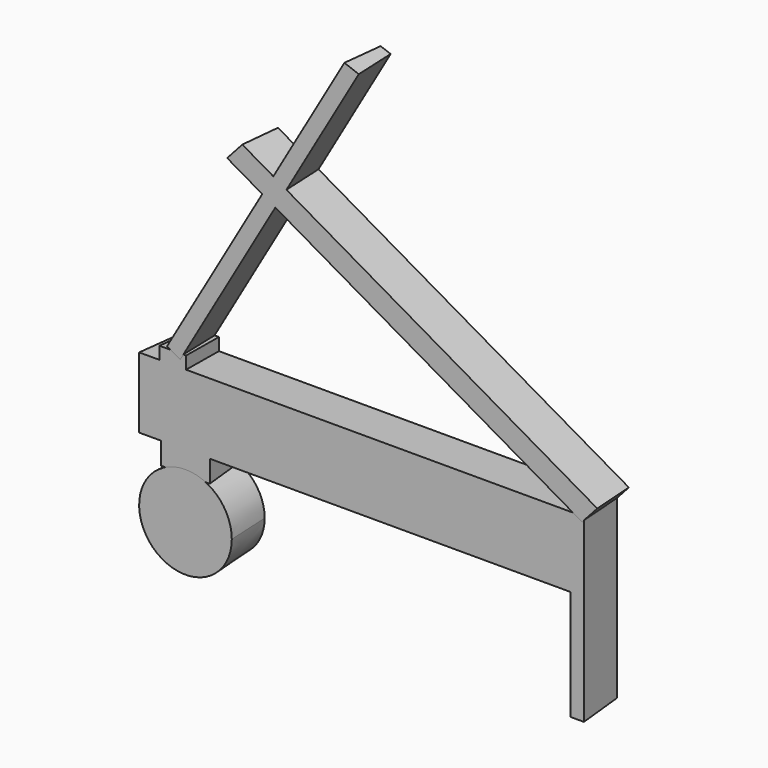
from build123d import *

# Parameters (mm, degrees)
F0_W                     = 5.08
F0_H                     = 63.5
F1_DEPTH                 = 25.4
DRAFT_F1_DRAFTED_ANGLE   = -3
DRAFT_F1_2_DRAFTED_ANGLE = -3
DRAFT_F1_3_DRAFTED_ANGLE = -3


# Not quite as in the source:
# - an extrude with a draft is written as a straight extrude whose walls are then drafted


with BuildPart() as f1:
    # F0 (on Front) → F1 (new body)
    with BuildSketch(Plane.XZ):
        Polygon((-170.315826494, -89.0998702904), (-170.315826494, -127.1998702904), (-157.615826494, -127.1998702904), (-132.215826494, -127.1998702904), (-127.624448756, -127.1998702904), (-102.224448756, -127.1998702904), (78.604173506, -127.1998702904), (83.684173506, -127.1998702904), (83.684173506, -89.0998702904), (-145.9128750829, -89.0998702904), (-158.6128750829, -89.0998702904), align=None)
        Polygon((-158.6128750829, -81.9087845771), (-158.6128750829, -89.0998702904), (-145.9128750829, -89.0998702904), (-145.9128750829, -81.9087845771), (-148.4528750829, -81.9087845771), align=None)
        Polygon((-132.215826494, -127.1998702904), (-157.615826494, -127.1998702904), (-157.615826494, -139.8998702904), (-144.915826494, -139.8998702904), (-132.215826494, -139.8998702904), align=None)
        with Locations((81.144173506, -158.9498702904)):
            Rectangle(F0_W, F0_H)
    extrude(amount=F1_DEPTH)

    # draft_F1_drafted
    draft_f1_drafted_walls = [f1.faces().sort_by_distance(p)[0] for p in [
        (-31.1143507884, -16.9333333333, -89.0998702904),
        (-145.9128750829, -16.9333333333, -85.5043274337),
        (-152.2628750829, -16.9333333333, -81.9087845771),
        (-158.6128750829, -16.9333333333, -85.5043274337),
        (-164.4643507884, -16.9333333333, -89.0998702904),
        (-170.315826494, -16.9333333333, -108.1498702904),
        (-163.965826494, -16.9333333333, -127.1998702904),
        (-157.615826494, -16.9333333333, -133.5498702904),
        (-144.915826494, -16.9333333333, -139.8998702904),
        (-132.215826494, -16.9333333333, -133.5498702904),
        (-26.805826494, -16.9333333333, -127.1998702904),
        (78.604173506, -16.9333333333, -158.9498702904),
        (81.144173506, -16.9333333333, -190.6998702904),
        (83.684173506, -16.9333333333, -139.8998702904),
    ]]
    draft(draft_f1_drafted_walls, neutral_plane=Plane.XZ, angle=DRAFT_F1_DRAFTED_ANGLE)


with BuildPart() as f1_2:
    # F0 (on Front) → F1, piece 2 (new body)
    with BuildSketch(Plane.XZ):
        Polygon((-153.7065332121, -78.875583642), (-148.4528750829, -81.9087845771), (-93.5324443899, 13.2161917567), (-98.7861025191, 16.2493926918), align=None)
        Polygon((-93.5324443899, 13.2161917567), (83.684173506, -89.0998702904), (90.6167230293, -81.4265449606), (-88.4766596756, 21.9730677541), align=None)
        Polygon((-118.7849083693, 27.7957086329), (-98.7861025191, 16.2493926918), (-93.7303178047, 25.0062686892), (-111.852358846, 35.4690339627), align=None)
        Polygon((-93.7303178047, 25.0062686892), (-88.4766596756, 21.9730677541), (-46.8528750829, 94.0675774719), (-52.6213717132, 96.2090519652), align=None)
        Polygon((-98.7861025191, 16.2493926918), (-93.5324443899, 13.2161917567), (-88.4766596756, 21.9730677541), (-93.7303178047, 25.0062686892), align=None)
    extrude(amount=F1_DEPTH)

    # draft_F1_2_drafted
    draft_f1_2_drafted_walls = [f1_2.faces().sort_by_distance(p)[0] for p in [
        (-151.0797041475, -16.9333333333, -80.3921841095),
        (-120.9926597364, -16.9333333333, -34.3462964102),
        (-4.9241354419, -16.9333333333, -37.9418392668),
        (87.1504482677, -16.9333333333, -85.2632076255),
        (1.0700316769, -16.9333333333, -29.7267386032),
        (-67.6647673792, -16.9333333333, 58.020322613),
        (-49.7371233981, -16.9333333333, 95.1383147186),
        (-73.175844759, -16.9333333333, 60.6076603272),
        (-102.7913383254, -16.9333333333, 30.237651326),
        (-115.3186336077, -16.9333333333, 31.6323712978),
        (-108.7855054442, -16.9333333333, 22.0225506624),
        (-126.2463178656, -16.9333333333, -31.3130954751),
    ]]
    draft(draft_f1_2_drafted_walls, neutral_plane=Plane.XZ, angle=DRAFT_F1_2_DRAFTED_ANGLE)


with BuildPart() as f1_3:
    # F0 (on Front) → F1, piece 3 (new body)
    with BuildSketch(Plane.XZ):
        with BuildLine():
            ThreePointArc((-119.515826494, -165.2998702904), (-126.9553142518, -147.3393580482), (-144.915826494, -139.8998702904))
            ThreePointArc((-144.915826494, -139.8998702904), (-162.8763387361, -183.2603825325), (-119.515826494, -165.2998702904))
        make_face()
    extrude(amount=F1_DEPTH)

    # draft_F1_3_drafted
    draft_f1_3_drafted_walls = [f1_3.faces().sort_by_distance(p)[0] for p in [
        (-170.315826494, -16.9333333333, -165.2998702904),
    ]]
    draft(draft_f1_3_drafted_walls, neutral_plane=Plane.XZ, angle=DRAFT_F1_3_DRAFTED_ANGLE)


solid = Compound([f1.part, f1_2.part, f1_3.part])
